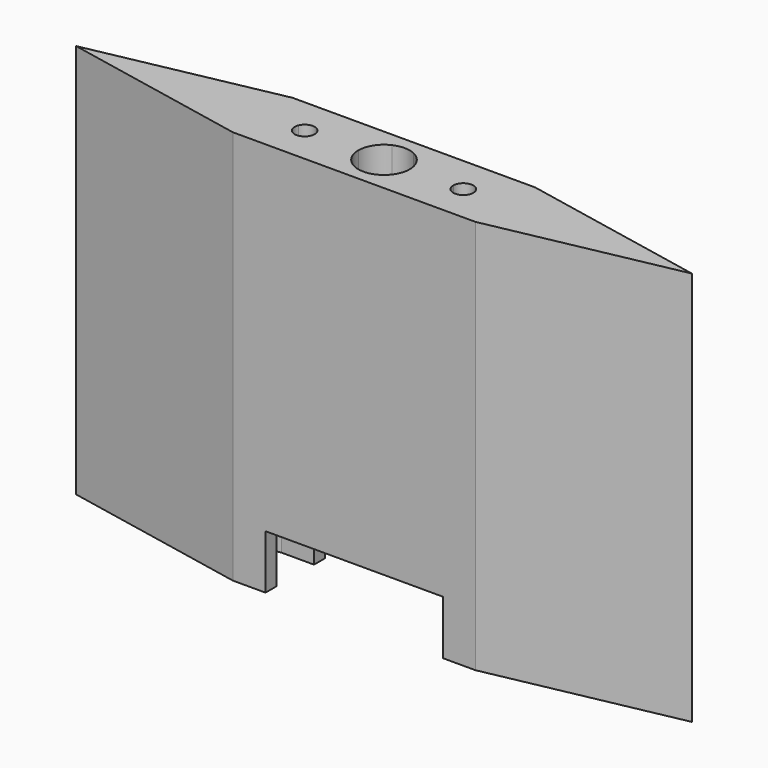
from build123d import *

# Parameters (mm, degrees)
F0_W     = 3.5
F0_H     = 1.5
F1_DEPTH = 35
F2_DEPTH = 1.5
F3_SIZE  = 1
F4_DEPTH = 7.3


with BuildPart() as f1:
    # F0 (on Top) → F1 (new body)
    with BuildSketch(Plane.XY):
        with BuildLine():
            ThreePointArc((-9.5, 0.394493346), (-8.2992202699, 1.0560835668), (-7.425, 0))
            Line((-7.425, 0), (-2.75, 0))
            ThreePointArc((-2.75, 0), (-2.314413618, 1.4852574204), (-1.1456439237, 2.5))
            Line((-1.1456439237, 2.5), (-9.5, 2.5))
            Line((-9.5, 2.5), (-9.5, 0.394493346))
        make_face()
        with BuildLine():
            ThreePointArc((-9.5, -0.394493346), (-9.575, 0), (-9.5, 0.394493346))
            Line((-9.5, 0.394493346), (-9.5, 2.5))
            Line((-9.5, 2.5), (-13, 2.5))
            Line((-13, 2.5), (-13, 0))
            Line((-13, 0), (-13, -2.5))
            Line((-13, -2.5), (-9.5, -2.5))
            Line((-9.5, -2.5), (-9.5, -0.394493346))
        make_face()
        with BuildLine():
            Line((-2.75, 0), (-7.425, 0))
            ThreePointArc((-7.425, 0), (-8.2992202699, -1.0560835668), (-9.5, -0.394493346))
            Line((-9.5, -0.394493346), (-9.5, -2.5))
            Line((-9.5, -2.5), (-1.1456439237, -2.5))
            ThreePointArc((-1.1456439237, -2.5), (-2.314413618, -1.4852574204), (-2.75, 0))
        make_face()
        Polygon((-13, -4), (-13, -2.5), (-25.5, 0), (-33, 0), align=None)
        Polygon((-25.5, 0), (-13, 2.5), (-13, 4), (-33, 0), align=None)
        Polygon((13, -2.5), (13, -4), (33, 0), (25.5, 0), align=None)
        Polygon((33, 0), (13, 4), (13, 2.5), (25.5, 0), align=None)
        Polygon((-25.5, 0), (-13, -2.5), (-13, 0), align=None)
        Polygon((-13, 0), (-13, 2.5), (-25.5, 0), align=None)
        with Locations((-11.25, 3.25)):
            Rectangle(F0_W, F0_H)
        with BuildLine():
            Line((-9.5, 4), (-9.5, 2.5))
            Line((-9.5, 2.5), (-1.1456439237, 2.5))
            ThreePointArc((-1.1456439237, 2.5), (0, 2.75), (1.1456439237, 2.5))
            Line((1.1456439237, 2.5), (9.5, 2.5))
            Line((9.5, 2.5), (9.5, 4))
            Line((9.5, 4), (-9.5, 4))
        make_face()
        with Locations((11.25, 3.25)):
            Rectangle(F0_W, F0_H)
        with Locations((11.25, -3.25)):
            Rectangle(F0_W, F0_H)
        with BuildLine():
            Line((-1.1456439237, -2.5), (-9.5, -2.5))
            Line((-9.5, -2.5), (-9.5, -4))
            Line((-9.5, -4), (9.5, -4))
            Line((9.5, -4), (9.5, -2.5))
            Line((9.5, -2.5), (1.1456439237, -2.5))
            ThreePointArc((1.1456439237, -2.5), (0, -2.75), (-1.1456439237, -2.5))
        make_face()
        with Locations((-11.25, -3.25)):
            Rectangle(F0_W, F0_H)
        Polygon((13, 0), (13, -2.5), (25.5, 0), align=None)
        Polygon((25.5, 0), (13, 2.5), (13, 0), align=None)
        with BuildLine():
            Line((9.5, 2.5), (9.5, 0.394493346))
            ThreePointArc((9.5, 0.394493346), (9.5560835668, 0.2007797301), (9.575, 0))
            ThreePointArc((9.575, 0), (9.5560835668, -0.2007797301), (9.5, -0.394493346))
            Line((9.5, -0.394493346), (9.5, -2.5))
            Line((9.5, -2.5), (13, -2.5))
            Line((13, -2.5), (13, 0))
            Line((13, 0), (13, 2.5))
            Line((13, 2.5), (9.5, 2.5))
        make_face()
        with BuildLine():
            ThreePointArc((1.1456439237, 2.5), (2.314413618, 1.4852574204), (2.75, 0))
            Line((2.75, 0), (7.425, 0))
            ThreePointArc((7.425, 0), (8.2992202699, 1.0560835668), (9.5, 0.394493346))
            Line((9.5, 0.394493346), (9.5, 2.5))
            Line((9.5, 2.5), (1.1456439237, 2.5))
        make_face()
        with BuildLine():
            Line((7.425, 0), (2.75, 0))
            ThreePointArc((2.75, 0), (2.314413618, -1.4852574204), (1.1456439237, -2.5))
            Line((1.1456439237, -2.5), (9.5, -2.5))
            Line((9.5, -2.5), (9.5, -0.394493346))
            ThreePointArc((9.5, -0.394493346), (8.2992202699, -1.0560835668), (7.425, 0))
        make_face()
    extrude(amount=F1_DEPTH)

    # F0 (on Top) → F2 (join)
    with BuildSketch(Plane.XY):
        Polygon((-13, -4), (-13, -2.5), (-25.5, 0), (-33, 0), align=None)
        Polygon((-25.5, 0), (-13, 2.5), (-13, 4), (-33, 0), align=None)
        with Locations((-11.25, 3.25)):
            Rectangle(F0_W, F0_H)
        with BuildLine():
            Line((-9.5, 4), (-9.5, 2.5))
            Line((-9.5, 2.5), (-1.1456439237, 2.5))
            ThreePointArc((-1.1456439237, 2.5), (0, 2.75), (1.1456439237, 2.5))
            Line((1.1456439237, 2.5), (9.5, 2.5))
            Line((9.5, 2.5), (9.5, 4))
            Line((9.5, 4), (-9.5, 4))
        make_face()
        with Locations((11.25, 3.25)):
            Rectangle(F0_W, F0_H)
        Polygon((-13, 0), (-13, 2.5), (-25.5, 0), align=None)
        Polygon((-25.5, 0), (-13, -2.5), (-13, 0), align=None)
        with BuildLine():
            ThreePointArc((-9.5, 0.394493346), (-8.2992202699, 1.0560835668), (-7.425, 0))
            Line((-7.425, 0), (-2.75, 0))
            ThreePointArc((-2.75, 0), (-2.314413618, 1.4852574204), (-1.1456439237, 2.5))
            Line((-1.1456439237, 2.5), (-9.5, 2.5))
            Line((-9.5, 2.5), (-9.5, 0.394493346))
        make_face()
        with BuildLine():
            ThreePointArc((-9.5, -0.394493346), (-9.575, 0), (-9.5, 0.394493346))
            Line((-9.5, 0.394493346), (-9.5, 2.5))
            Line((-9.5, 2.5), (-13, 2.5))
            Line((-13, 2.5), (-13, 0))
            Line((-13, 0), (-13, -2.5))
            Line((-13, -2.5), (-9.5, -2.5))
            Line((-9.5, -2.5), (-9.5, -0.394493346))
        make_face()
        with BuildLine():
            Line((-2.75, 0), (-7.425, 0))
            ThreePointArc((-7.425, 0), (-8.2992202699, -1.0560835668), (-9.5, -0.394493346))
            Line((-9.5, -0.394493346), (-9.5, -2.5))
            Line((-9.5, -2.5), (-1.1456439237, -2.5))
            ThreePointArc((-1.1456439237, -2.5), (-2.314413618, -1.4852574204), (-2.75, 0))
        make_face()
        with Locations((11.25, -3.25)):
            Rectangle(F0_W, F0_H)
        with BuildLine():
            Line((-1.1456439237, -2.5), (-9.5, -2.5))
            Line((-9.5, -2.5), (-9.5, -4))
            Line((-9.5, -4), (9.5, -4))
            Line((9.5, -4), (9.5, -2.5))
            Line((9.5, -2.5), (1.1456439237, -2.5))
            ThreePointArc((1.1456439237, -2.5), (0, -2.75), (-1.1456439237, -2.5))
        make_face()
        with Locations((-11.25, -3.25)):
            Rectangle(F0_W, F0_H)
        Polygon((13, -2.5), (13, -4), (33, 0), (25.5, 0), align=None)
        Polygon((13, 0), (13, -2.5), (25.5, 0), align=None)
        Polygon((25.5, 0), (13, 2.5), (13, 0), align=None)
        Polygon((33, 0), (13, 4), (13, 2.5), (25.5, 0), align=None)
        with BuildLine():
            ThreePointArc((1.1456439237, 2.5), (2.314413618, 1.4852574204), (2.75, 0))
            Line((2.75, 0), (7.425, 0))
            ThreePointArc((7.425, 0), (8.2992202699, 1.0560835668), (9.5, 0.394493346))
            Line((9.5, 0.394493346), (9.5, 2.5))
            Line((9.5, 2.5), (1.1456439237, 2.5))
        make_face()
        with BuildLine():
            Line((7.425, 0), (2.75, 0))
            ThreePointArc((2.75, 0), (2.314413618, -1.4852574204), (1.1456439237, -2.5))
            Line((1.1456439237, -2.5), (9.5, -2.5))
            Line((9.5, -2.5), (9.5, -0.394493346))
            ThreePointArc((9.5, -0.394493346), (8.2992202699, -1.0560835668), (7.425, 0))
        make_face()
        with BuildLine():
            Line((9.5, 2.5), (9.5, 0.394493346))
            ThreePointArc((9.5, 0.394493346), (9.5560835668, 0.2007797301), (9.575, 0))
            ThreePointArc((9.575, 0), (9.5560835668, -0.2007797301), (9.5, -0.394493346))
            Line((9.5, -0.394493346), (9.5, -2.5))
            Line((9.5, -2.5), (13, -2.5))
            Line((13, -2.5), (13, 0))
            Line((13, 0), (13, 2.5))
            Line((13, 2.5), (9.5, 2.5))
        make_face()
    extrude(amount=-F2_DEPTH)

    # F3
    f3_edges = [f1.edges().sort_by_distance(p)[0] for p in [
        (-9.575, 0, -1.5),
        (7.5, -0.394493, -1.5),
        (1.145644, -2.5, -1.5),
    ]]
    chamfer(f3_edges, length=F3_SIZE)

    # F0 (on Top) → F4 (join)
    with BuildSketch(Plane.XY):
        with Locations((-11.25, 3.25)):
            Rectangle(F0_W, F0_H)
        with Locations((11.25, 3.25)):
            Rectangle(F0_W, F0_H)
        Polygon((-25.5, 0), (-13, 2.5), (-13, 4), (-33, 0), align=None)
        Polygon((-13, -4), (-13, -2.5), (-25.5, 0), (-33, 0), align=None)
        with Locations((11.25, -3.25)):
            Rectangle(F0_W, F0_H)
        with Locations((-11.25, -3.25)):
            Rectangle(F0_W, F0_H)
        Polygon((33, 0), (13, 4), (13, 2.5), (25.5, 0), align=None)
        Polygon((13, -2.5), (13, -4), (33, 0), (25.5, 0), align=None)
    extrude(amount=-F4_DEPTH)


solid = f1.part
